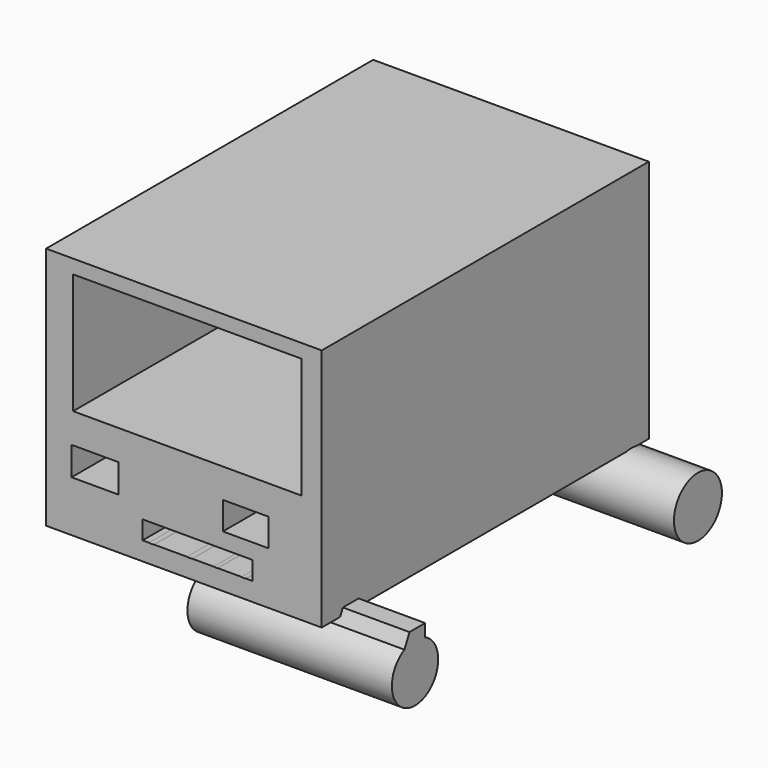
from build123d import *

# Parameters (mm, degrees)
F0_W     = 102.7466543019
F0_H     = 90.9466221929
F0_W_2   = 85.1905047894
F0_H_2   = 44.8976957705
F1_DEPTH = 152.4
F2_R     = 11.1763524663
F3_DEPTH = 76.2


with BuildPart() as f1:
    # F0 (on Front) → F1 (new body)
    with BuildSketch(Plane.XZ):
        with Locations((-1.8626e-06, 7.9146586359)):
            Rectangle(F0_W, F0_H)
        Polygon((-41.8757386506, -12.8073554952), (-41.8757386506, -7.9146586359), (-37.270847708, -7.9146586359), (-24.3195872754, -7.9146586359), (-24.3195872754, -18.5634717345), (-37.270847708, -18.5634717345), (-41.8757386506, -18.5634717345), align=None, mode=Mode.SUBTRACT)
        with BuildLine():
            Line((-15.3976082802, -30.6513141841), (-15.3976082802, -23.7439740449))
            Line((-15.3976082802, -23.7439740449), (25.5187885163, -23.7439740449))
            Line((25.5187885163, -23.7439740449), (25.5187885163, -30.6513141841))
            Line((25.5187885163, -30.6513141841), (23.2219085714, -30.6513141841))
            add(Edge.make_bspline(
                [(23.2219085714, -30.6513141841), (22.85194256, -30.745750475), (22.4083868695, -30.745750475)],
                knots=[0.6101406025, 0.6101406025, 0.6101406025, 1, 1, 1], degree=2))
            add(Edge.make_bspline(
                [(22.4083868695, -30.745750475), (21.9525027452, -30.745750475), (21.5799819799, -30.6513141841)],
                knots=[0, 0, 0, 0.4594075276, 0.4594075276, 0.4594075276], degree=2))
            Line((21.5799819799, -30.6513141841), (17.1949040127, -30.6513141841))
            Line((17.1949040127, -30.6513141841), (15.8233293106, -30.6513141841))
            Line((15.8233293106, -30.6513141841), (12.6383256981, -30.6513141841))
            add(Edge.make_bspline(
                [(12.6383256981, -30.6513141841), (12.2965846392, -30.745750475), (11.8839868875, -30.745750475)],
                knots=[0.6033851102, 0.6033851102, 0.6033851102, 1, 1, 1], degree=2))
            add(Edge.make_bspline(
                [(11.8839868875, -30.745750475), (11.4876624367, -30.745750475), (11.1537473039, -30.6513141841)],
                knots=[0, 0, 0, 0.3398387497, 0.3398387497, 0.3398387497], degree=2))
            Line((11.1537473039, -30.6513141841), (3.1983305145, -30.6513141841))
            add(Edge.make_bspline(
                [(3.1983305145, -30.6513141841), (2.7104556951, -30.745750475), (2.1975216142, -30.745750475)],
                knots=[0.4435987872, 0.4435987872, 0.4435987872, 1, 1, 1], degree=2))
            add(Edge.make_bspline(
                [(2.1975216142, -30.745750475), (1.6733949816, -30.745750475), (1.2280841955, -30.6513141841)],
                knots=[0, 0, 0, 0.325259052, 0.325259052, 0.325259052], degree=2))
            Line((1.2280841955, -30.6513141841), (-2.1870204663, -30.6513141841))
            Line((-2.1870204663, -30.6513141841), (-3.5690880896, -30.6513141841))
            Line((-3.5690880896, -30.6513141841), (-6.4456474922, -30.6513141841))
            Line((-6.4456474922, -30.6513141841), (-7.8277151155, -30.6513141841))
            Line((-7.8277151155, -30.6513141841), (-11.0580714674, -30.6513141841))
            add(Edge.make_bspline(
                [(-11.0580714674, -30.6513141841), (-11.4916109594, -30.745750475), (-12.0113927042, -30.745750475)],
                knots=[0.6303252294, 0.6303252294, 0.6303252294, 1, 1, 1], degree=2))
            add(Edge.make_bspline(
                [(-12.0113927042, -30.745750475), (-12.5246569888, -30.745750475), (-12.9473134807, -30.6513141841)],
                knots=[0, 0, 0, 0.3766854018, 0.3766854018, 0.3766854018], degree=2))
            Line((-12.9473134807, -30.6513141841), (-15.3976082802, -30.6513141841))
        make_face(mode=Mode.SUBTRACT)
        Polygon((14.5341921598, -17.9878585041), (14.5341921598, -7.6268524863), (26.0464195162, -7.6268524863), (31.5147265792, -7.6268524863), (31.5147265792, -12.8073554952), (31.5147265792, -17.9878585041), (26.0464195162, -17.9878585041), align=None, mode=Mode.SUBTRACT)
        with Locations((1.2951269746, 25.7586139487)):
            Rectangle(F0_W_2, F0_H_2, mode=Mode.SUBTRACT)
    extrude(amount=F1_DEPTH)

    # F2 (on Right) → F3 (join)
    with BuildSketch(Plane.YZ):
        with Locations((-8.1405537203, -48.4952703118)):
            Circle(F2_R)
        with BuildLine():
            ThreePointArc((-144.905696857, -39.7735155561), (-145.56909186, -58.572575633), (-129.1690343005, -49.3593859167))
            ThreePointArc((-129.1690343005, -49.3593859167), (-130.8108710033, -43.6385160791), (-135.2366314328, -39.6589904693))
            ThreePointArc((-135.2366314328, -39.6589904693), (-140.084714499, -38.57223065), (-144.905696857, -39.7735155561))
        make_face()
        with BuildLine():
            ThreePointArc((-144.905696857, -39.7735155561), (-140.084714499, -38.57223065), (-135.2366314328, -39.6589904693))
            Line((-135.2366314328, -39.6589904693), (-135.2366314328, -34.9684022367))
            Line((-135.2366314328, -34.9684022367), (-142.5458490849, -34.9684022367))
            Line((-142.5458490849, -34.9684022367), (-144.905696857, -39.7735155561))
        make_face()
    extrude(amount=F3_DEPTH)


solid = f1.part
